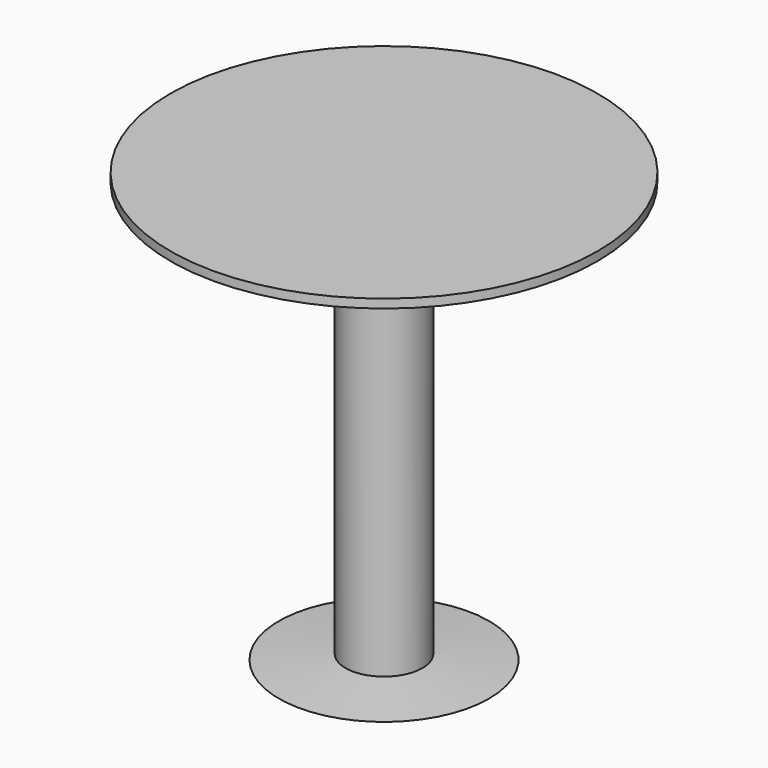
from build123d import *

# Parameters (mm, degrees)
F0_R     = 110
F1_DEPTH = 1200
F2_R     = 609.6
F2_R_2   = 110
F3_DEPTH = 25
F4_R     = 300
F4_R_2   = 110
F5_DEPTH = 15
F6_SIZE2 = 189.99999
F6_SIZE  = 14.99999


# Not quite as in the source:
# - a fillet or chamfer is up to 0.001 mm smaller than in the source, because OpenCascade refuses the exact size


with BuildPart() as f1:
    # F0 (on Top) → F1 (new body)
    with BuildSketch(Plane.XY):
        Circle(F0_R)
    extrude(amount=F1_DEPTH)

    # F2 (on face) → F3 (join)
    with BuildSketch(Plane.XY.offset(1200)):
        Circle(F2_R)
        Circle(F2_R_2, mode=Mode.SUBTRACT)
        Circle(F2_R_2)
    extrude(amount=F3_DEPTH)

    # F4 (on face) → F5 (join)
    with BuildSketch(Plane(origin=(0, 0, 0), x_dir=(1, 0, 0), z_dir=(0, 0, -1))):
        Circle(F4_R)
        Circle(F4_R_2, mode=Mode.SUBTRACT)
    extrude(amount=-F5_DEPTH)

    # F6 (size 15 and 190 in the source; OpenCascade refuses exactly that, so slightly less here)
    f6_edges = [f1.edges().sort_by_distance(p)[0] for p in [
        (-300, 0, 15),
    ]]
    f6_side = f1.faces().sort_by_distance((-300, 0, 7.5))[0]
    chamfer(f6_edges, length=F6_SIZE, length2=F6_SIZE2, reference=f6_side)


solid = f1.part
